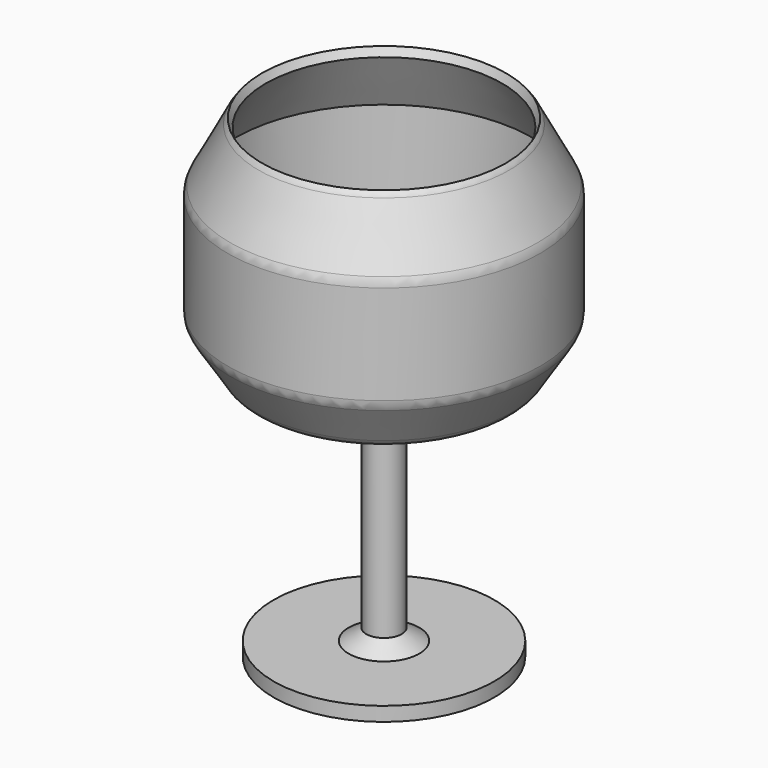
from build123d import *

# Parameters (mm, degrees)
F3_R = 5.08
F4_R = 5.08
F5_R = 5.08


# Not quite as in the source:
# - a fillet or chamfer that OpenCascade refuses, or shapes differently, is made with other operations: its cross-section is extruded or revolved along the edge and cut away or added


with BuildPart() as f1:
    # F0 (on Front) → F1 (revolve)
    with BuildSketch(Plane.XZ):
        Polygon((-31.5286010422, 51.7711788416), (-32.5126800885, 53.8890883327), (-32.7099710703, 53.8890883327), (-41.6522659361, 36.9457937777), (-41.6522659361, 7.7656768262), (-32.7099710703, -6.3537354581), (-12.7074699849, -6.3537354581), (-4.7064702958, -6.3537354581), (-4.7064702958, -65.6552687287), (-9.4129405916, -68.7144696712), (-29.415441677, -68.7144696712), (-29.415441677, -72.4796503782), (0, -72.4796503782), (0, -4.3968333285), (-12.472147122, -4.3968333285), (-31.5333530307, -4.3968333285), (-39.5343527198, 8.2363234833), (-39.5343527198, 36.475148052), (-31.5333530307, 51.7711788416), align=None)
    revolve(axis=Axis((0, 0, -0.3529824317), (0, 0, -1)))

    # F2: fillet of radius 7.62 on 1 edges, made by hand

    # F2_s1 → F2_t2 (revolve, cut)
    with BuildSketch(Plane.XZ):
        with BuildLine():
            ThreePointArc((-32.5126800885, 53.8890883327), (-33.0044959985, 53.2373184877), (-33.4237493814, 52.5366663478))
            Line((-33.4237493814, 52.5366663478), (-32.7099710703, 53.8890883327))
            Line((-32.7099710703, 53.8890883327), (-32.5126800885, 53.8890883327))
        make_face()
    revolve(axis=Axis((0, 0, 53.8890883327), (0, 0, -1)), mode=Mode.SUBTRACT)

    # F3
    f3_edges = [f1.edges().sort_by_distance(p)[0] for p in [
        (41.652266, 0, 36.945794),
    ]]
    fillet(f3_edges, radius=F3_R)

    # F4
    f4_edges = [f1.edges().sort_by_distance(p)[0] for p in [
        (41.652266, 0, 7.765677),
    ]]
    fillet(f4_edges, radius=F4_R)

    # F5
    f5_edges = [f1.edges().sort_by_distance(p)[0] for p in [
        (32.709971, 0, -6.353735),
    ]]
    fillet(f5_edges, radius=F5_R)


solid = f1.part
